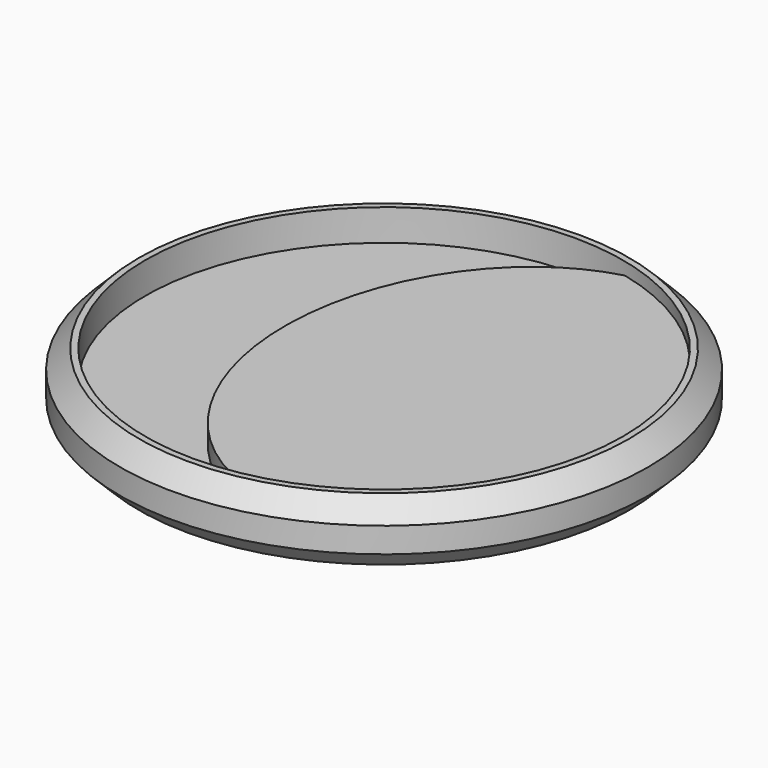
from build123d import *

# Parameters (mm, degrees)
F0_R          = 10
F1_DEPTH      = 1.5
F3_DEPTH      = 0.75
F4_R          = 10.5
F4_R_2        = 9.5
F5_DEPTH      = 2
F5_DEPTH_BACK = 0.5
F6_SIZE       = 0.75


# Not quite as in the source:
# - a feature of the source that left no trace in its solid (it failed there, or was rolled back) is left out


with BuildPart() as f1:
    # F0 (on Top) → F1 (new body)
    with BuildSketch(Plane.XY):
        Circle(F0_R)
    extrude(amount=F1_DEPTH)

    # F2 (on face) → F3 (cut)
    with BuildSketch(Plane.XY.offset(1.5)):
        with BuildLine():
            add(Edge.make_bspline(
                [(3.2873270655, 9.444230025), (-3.9457486769, 8.7871247234), (-3.9457486769, 0), (-3.9457486769, -8.7871247234), (3.2873270655, -9.444230025)],
                knots=[0.0748503411, 0.0748503411, 0.0748503411, 1.5707963268, 1.5707963268, 3.0667423125, 3.0667423125, 3.0667423125], degree=2, weights=[1, 0.7330690514, 1, 0.7330690514, 1]))
            ThreePointArc((3.2873270655, 9.444230025), (-10, 0), (3.2873270655, -9.444230025))
        make_face()
    extrude(amount=-F3_DEPTH, mode=Mode.SUBTRACT)

    # F4 (on Top) → F5 (join, two sides)
    with BuildSketch(Plane.XY) as f5_sk:
        Circle(F4_R)
        Circle(F4_R_2, mode=Mode.SUBTRACT)
    extrude(amount=F5_DEPTH)
    extrude(f5_sk.sketch, amount=-F5_DEPTH_BACK)

    # F6
    f6_edges = [f1.edges().sort_by_distance(p)[0] for p in [
        (-10.5, 0, 2),
        (-10.5, 0, -0.5),
    ]]
    chamfer(f6_edges, length=F6_SIZE)


solid = f1.part
